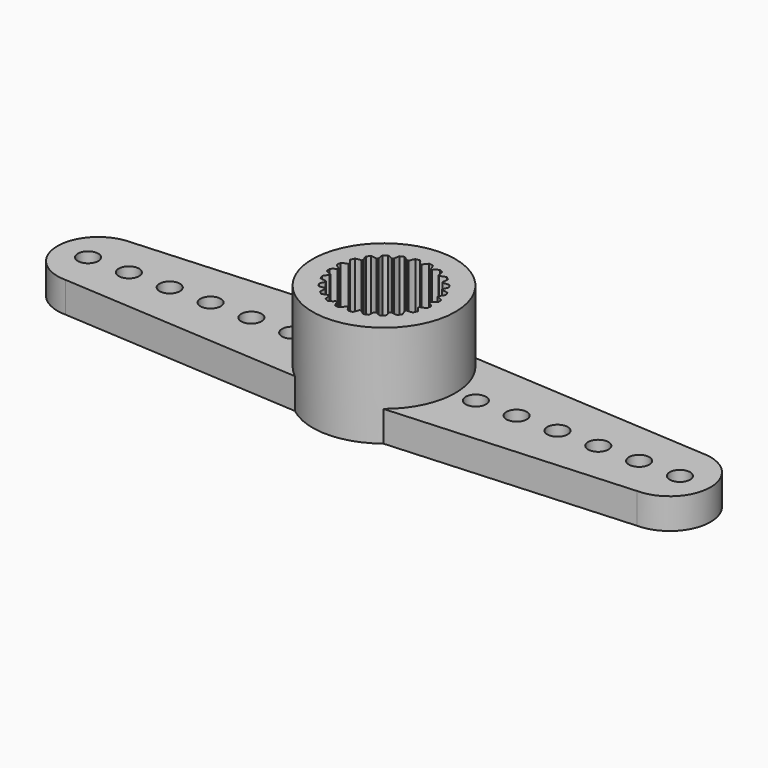
from build123d import *

# Parameters (mm, degrees)
F0_R     = 0.5
F0_R_2   = 1
F1_DEPTH = 1.5
F2_DEPTH = 5
F3_R     = 2.375
F4_DEPTH = 1
F6_DEPTH = 2.75


# Not quite as in the source:
# - a feature names something its author has since deleted; it is built from what else it names


with BuildPart() as f1:
    # F0 (on Top) → F1 (new body)
    with BuildSketch(Plane.XY):
        with BuildLine():
            ThreePointArc((-2.1650635095, -2.75), (-3.5, 0), (-2.1650635095, 2.75))
            Line((-2.1650635095, 2.75), (-14, 2))
            ThreePointArc((-14, 2), (-12.5857864376, 1.4142135624), (-12, 0))
            ThreePointArc((-12, 0), (-12.5857864376, -1.4142135624), (-14, -2))
            Line((-14, -2), (-2.1650635095, -2.75))
        make_face()
        with Locations((-10.5, 0)):
            Circle(F0_R, mode=Mode.SUBTRACT)
        with Locations((-8.5, 0)):
            Circle(F0_R, mode=Mode.SUBTRACT)
        with Locations((-6.5, 0)):
            Circle(F0_R, mode=Mode.SUBTRACT)
        with Locations((-4.5, 0)):
            Circle(F0_R, mode=Mode.SUBTRACT)
        with BuildLine():
            ThreePointArc((-2.1650635095, -2.75), (1.5284432794, -3.148628454), (3.5, 0))
            ThreePointArc((3.5, 0), (1.5284432794, 3.148628454), (-2.1650635095, 2.75))
            ThreePointArc((-2.1650635095, 2.75), (-3.5, 0), (-2.1650635095, -2.75))
        make_face()
        Circle(F0_R_2, mode=Mode.SUBTRACT)
        with BuildLine():
            ThreePointArc((-12, 0), (-12.5857864376, 1.4142135624), (-14, 2))
            ThreePointArc((-14, 2), (-16, 0), (-14, -2))
            ThreePointArc((-14, -2), (-12.5857864376, -1.4142135624), (-12, 0))
        make_face()
        with Locations((-14.5, 0)):
            Circle(F0_R, mode=Mode.SUBTRACT)
        with Locations((-12.5, 0)):
            Circle(F0_R, mode=Mode.SUBTRACT)
    extrude(amount=F1_DEPTH)

    # F0 (on Top) → F2 (join)
    with BuildSketch(Plane.XY):
        with BuildLine():
            ThreePointArc((-2.1650635095, -2.75), (1.5284432794, -3.148628454), (3.5, 0))
            ThreePointArc((3.5, 0), (1.5284432794, 3.148628454), (-2.1650635095, 2.75))
            ThreePointArc((-2.1650635095, 2.75), (-3.5, 0), (-2.1650635095, -2.75))
        make_face()
        Circle(F0_R_2, mode=Mode.SUBTRACT)
    extrude(amount=F2_DEPTH)

    # F3 (on face) → F4 (cut)
    with BuildSketch(Plane.XY):
        Circle(F3_R)
    extrude(amount=F4_DEPTH, mode=Mode.SUBTRACT)

    # F5 (on face) → F6 (cut)
    with BuildSketch(Plane.XY.offset(5)):
        with BuildLine():
            ThreePointArc((2.2496444163, -0.04), (2.2499111023, -0.0200007902), (2.25, 0))
            ThreePointArc((2.25, 0), (2.2499111023, 0.0200007902), (2.2496444163, 0.04))
            ThreePointArc((2.2496444163, 0.04), (2.2307509381, 0.2936839325), (2.1833424035, 0.5436137866))
            ThreePointArc((2.1833424035, 0.5436137866), (2.1733331092, 0.5823428515), (2.1626368799, 0.6208878527))
            ThreePointArc((2.1626368799, 0.6208878527), (2.0787289482, 0.8610377228), (1.968249214, 1.090181192))
            ThreePointArc((1.968249214, 1.090181192), (1.9485571585, 1.125), (1.928249214, 1.1594632243))
            ThreePointArc((1.928249214, 1.1594632243), (1.7850450157, 1.3697132153), (1.6190230933, 1.5624545508))
            ThreePointArc((1.6190230933, 1.5624545508), (1.5909902577, 1.5909902577), (1.5624545508, 1.6190230933))
            ThreePointArc((1.5624545508, 1.6190230933), (1.3697132153, 1.7850450157), (1.1594632243, 1.928249214))
            ThreePointArc((1.1594632243, 1.928249214), (1.125, 1.9485571585), (1.090181192, 1.968249214))
            ThreePointArc((1.090181192, 1.968249214), (0.8610377228, 2.0787289482), (0.6208878527, 2.1626368799))
            ThreePointArc((0.6208878527, 2.1626368799), (0.5823428515, 2.1733331092), (0.5436137866, 2.1833424035))
            ThreePointArc((0.5436137866, 2.1833424035), (0.2936839325, 2.2307509381), (0.04, 2.2496444163))
            ThreePointArc((0.04, 2.2496444163), (0, 2.25), (-0.04, 2.2496444163))
            ThreePointArc((-0.04, 2.2496444163), (-0.2936839325, 2.2307509381), (-0.5436137866, 2.1833424035))
            ThreePointArc((-0.5436137866, 2.1833424035), (-0.5823428515, 2.1733331092), (-0.6208878527, 2.1626368799))
            ThreePointArc((-0.6208878527, 2.1626368799), (-0.8610377228, 2.0787289482), (-1.090181192, 1.968249214))
            ThreePointArc((-1.090181192, 1.968249214), (-1.125, 1.9485571585), (-1.1594632243, 1.928249214))
            ThreePointArc((-1.1594632243, 1.928249214), (-1.3697132153, 1.7850450157), (-1.5624545508, 1.6190230933))
            ThreePointArc((-1.5624545508, 1.6190230933), (-1.5909902577, 1.5909902577), (-1.6190230933, 1.5624545508))
            ThreePointArc((-1.6190230933, 1.5624545508), (-1.7850450157, 1.3697132153), (-1.928249214, 1.1594632243))
            ThreePointArc((-1.928249214, 1.1594632243), (-1.9485571585, 1.125), (-1.968249214, 1.090181192))
            ThreePointArc((-1.968249214, 1.090181192), (-2.0787289482, 0.8610377228), (-2.1626368799, 0.6208878527))
            ThreePointArc((-2.1626368799, 0.6208878527), (-2.1733331092, 0.5823428515), (-2.1833424035, 0.5436137866))
            ThreePointArc((-2.1833424035, 0.5436137866), (-2.2307509381, 0.2936839325), (-2.2496444163, 0.04))
            ThreePointArc((-2.2496444163, 0.04), (-2.25, 0), (-2.2496444163, -0.04))
            ThreePointArc((-2.2496444163, -0.04), (-2.2307509381, -0.2936839325), (-2.1833424035, -0.5436137866))
            ThreePointArc((-2.1833424035, -0.5436137866), (-2.1733331092, -0.5823428515), (-2.1626368799, -0.6208878527))
            ThreePointArc((-2.1626368799, -0.6208878527), (-2.0787289482, -0.8610377228), (-1.968249214, -1.090181192))
            ThreePointArc((-1.968249214, -1.090181192), (-1.9485571585, -1.125), (-1.928249214, -1.1594632243))
            ThreePointArc((-1.928249214, -1.1594632243), (-1.7850450157, -1.3697132153), (-1.6190230933, -1.5624545508))
            ThreePointArc((-1.6190230933, -1.5624545508), (-1.5909902577, -1.5909902577), (-1.5624545508, -1.6190230933))
            ThreePointArc((-1.5624545508, -1.6190230933), (-1.3697132153, -1.7850450157), (-1.1594632243, -1.928249214))
            ThreePointArc((-1.1594632243, -1.928249214), (-1.125, -1.9485571585), (-1.090181192, -1.968249214))
            ThreePointArc((-1.090181192, -1.968249214), (-0.8610377228, -2.0787289482), (-0.6208878527, -2.1626368799))
            ThreePointArc((-0.6208878527, -2.1626368799), (-0.5823428515, -2.1733331092), (-0.5436137866, -2.1833424035))
            ThreePointArc((-0.5436137866, -2.1833424035), (-0.2936839325, -2.2307509381), (-0.04, -2.2496444163))
            ThreePointArc((-0.04, -2.2496444163), (0, -2.25), (0.04, -2.2496444163))
            ThreePointArc((0.04, -2.2496444163), (0.2936839325, -2.2307509381), (0.5436137866, -2.1833424035))
            ThreePointArc((0.5436137866, -2.1833424035), (0.5823428515, -2.1733331092), (0.6208878527, -2.1626368799))
            ThreePointArc((0.6208878527, -2.1626368799), (0.8610377228, -2.0787289482), (1.090181192, -1.968249214))
            ThreePointArc((1.090181192, -1.968249214), (1.125, -1.9485571585), (1.1594632243, -1.928249214))
            ThreePointArc((1.1594632243, -1.928249214), (1.3697132153, -1.7850450157), (1.5624545508, -1.6190230933))
            ThreePointArc((1.5624545508, -1.6190230933), (1.5909902577, -1.5909902577), (1.6190230933, -1.5624545508))
            ThreePointArc((1.6190230933, -1.5624545508), (1.7850450157, -1.3697132153), (1.928249214, -1.1594632243))
            ThreePointArc((1.928249214, -1.1594632243), (1.9485571585, -1.125), (1.968249214, -1.090181192))
            ThreePointArc((1.968249214, -1.090181192), (2.0787289482, -0.8610377228), (2.1626368799, -0.6208878527))
            ThreePointArc((2.1626368799, -0.6208878527), (2.1733331092, -0.5823428515), (2.1833424035, -0.5436137866))
            ThreePointArc((2.1833424035, -0.5436137866), (2.2307509381, -0.2936839325), (2.2496444163, -0.04))
        make_face()
        with BuildLine():
            ThreePointArc((2.1833424035, 0.5436137866), (2.2307509381, 0.2936839325), (2.2496444163, 0.04))
            ThreePointArc((2.2496444163, 0.04), (2.376347735, 0.1239325273), (2.4898544134, 0.225))
            ThreePointArc((2.4898544134, 0.225), (2.47674458, 0.3260696098), (2.4632489668, 0.4270884308))
            ThreePointArc((2.4632489668, 0.4270884308), (2.3313772515, 0.5047639091), (2.1833424035, 0.5436137866))
        make_face()
        with BuildLine():
            ThreePointArc((2.4898544134, -0.225), (2.382580011, -0.115840338), (2.2496444163, -0.04))
            ThreePointArc((2.2496444163, -0.04), (2.2307509381, -0.2936839325), (2.1833424035, -0.5436137866))
            ThreePointArc((2.1833424035, -0.5436137866), (2.3274517478, -0.4953344228), (2.4632489668, -0.4270884308))
            ThreePointArc((2.4632489668, -0.4270884308), (2.47674458, -0.3260696098), (2.4898544134, -0.225))
        make_face()
        with BuildLine():
            ThreePointArc((1.968249214, 1.090181192), (2.0787289482, 0.8610377228), (2.1626368799, 0.6208878527))
            ThreePointArc((2.1626368799, 0.6208878527), (2.2632995511, 0.7347536804), (2.3467803965, 0.8617550526))
            ThreePointArc((2.3467803965, 0.8617550526), (2.3079585298, 0.9559877245), (2.2687771737, 1.0500714909))
            ThreePointArc((2.2687771737, 1.0500714909), (2.1212949851, 1.09096933), (1.968249214, 1.090181192))
        make_face()
        with BuildLine():
            ThreePointArc((2.3467803965, -0.8617550526), (2.2714138802, -0.7285502576), (2.1626368799, -0.6208878527))
            ThreePointArc((2.1626368799, -0.6208878527), (2.0787289482, -0.8610377228), (1.968249214, -1.090181192))
            ThreePointArc((1.968249214, -1.090181192), (2.1199437704, -1.0808451505), (2.2687771737, -1.0500714909))
            ThreePointArc((2.2687771737, -1.0500714909), (2.3079585298, -0.9559877245), (2.3467803965, -0.8617550526))
        make_face()
        with BuildLine():
            ThreePointArc((1.6190230933, 1.5624545508), (1.7850450157, 1.3697132153), (1.928249214, 1.1594632243))
            ThreePointArc((1.928249214, 1.1594632243), (1.9960112431, 1.2955025845), (2.0437771737, 1.4397829226))
            ThreePointArc((2.0437771737, 1.4397829226), (1.98188892, 1.5207568555), (1.9196919657, 1.6014939141))
            ThreePointArc((1.9196919657, 1.6014939141), (1.7666499711, 1.602826994), (1.6190230933, 1.5624545508))
        make_face()
        with BuildLine():
            ThreePointArc((2.0437771737, -1.4397829226), (2.0054546471, -1.291610681), (1.928249214, -1.1594632243))
            ThreePointArc((1.928249214, -1.1594632243), (1.7850450157, -1.3697132153), (1.6190230933, -1.5624545508))
            ThreePointArc((1.6190230933, -1.5624545508), (1.7679651283, -1.5926980674), (1.9196919657, -1.6014939141))
            ThreePointArc((1.9196919657, -1.6014939141), (1.98188892, -1.5207568555), (2.0437771737, -1.4397829226))
        make_face()
        with BuildLine():
            ThreePointArc((1.1594632243, 1.928249214), (1.3697132153, 1.7850450157), (1.5624545508, 1.6190230933))
            ThreePointArc((1.5624545508, 1.6190230933), (1.5926980674, 1.7679651283), (1.6014939141, 1.9196919657))
            ThreePointArc((1.6014939141, 1.9196919657), (1.5207568555, 1.98188892), (1.4397829226, 2.0437771737))
            ThreePointArc((1.4397829226, 2.0437771737), (1.291610681, 2.0054546471), (1.1594632243, 1.928249214))
        make_face()
        with BuildLine():
            ThreePointArc((1.6014939141, -1.9196919657), (1.602826994, -1.7666499711), (1.5624545508, -1.6190230933))
            ThreePointArc((1.5624545508, -1.6190230933), (1.3697132153, -1.7850450157), (1.1594632243, -1.928249214))
            ThreePointArc((1.1594632243, -1.928249214), (1.2955025845, -1.9960112431), (1.4397829226, -2.0437771737))
            ThreePointArc((1.4397829226, -2.0437771737), (1.5207568555, -1.98188892), (1.6014939141, -1.9196919657))
        make_face()
        with BuildLine():
            ThreePointArc((0.6208878527, 2.1626368799), (0.8610377228, 2.0787289482), (1.090181192, 1.968249214))
            ThreePointArc((1.090181192, 1.968249214), (1.0808451505, 2.1199437704), (1.0500714909, 2.2687771737))
            ThreePointArc((1.0500714909, 2.2687771737), (0.9559877245, 2.3079585298), (0.8617550526, 2.3467803965))
            ThreePointArc((0.8617550526, 2.3467803965), (0.7285502576, 2.2714138802), (0.6208878527, 2.1626368799))
        make_face()
        with BuildLine():
            ThreePointArc((1.0500714909, -2.2687771737), (1.09096933, -2.1212949851), (1.090181192, -1.968249214))
            ThreePointArc((1.090181192, -1.968249214), (0.8610377228, -2.0787289482), (0.6208878527, -2.1626368799))
            ThreePointArc((0.6208878527, -2.1626368799), (0.7347536804, -2.2632995511), (0.8617550526, -2.3467803965))
            ThreePointArc((0.8617550526, -2.3467803965), (0.9559877245, -2.3079585298), (1.0500714909, -2.2687771737))
        make_face()
        with BuildLine():
            ThreePointArc((0.04, 2.2496444163), (0.2936839325, 2.2307509381), (0.5436137866, 2.1833424035))
            ThreePointArc((0.5436137866, 2.1833424035), (0.4953344228, 2.3274517478), (0.4270884308, 2.4632489668))
            ThreePointArc((0.4270884308, 2.4632489668), (0.3260696098, 2.47674458), (0.225, 2.4898544134))
            ThreePointArc((0.225, 2.4898544134), (0.115840338, 2.382580011), (0.04, 2.2496444163))
        make_face()
        with BuildLine():
            ThreePointArc((0.4270884308, -2.4632489668), (0.5047639091, -2.3313772515), (0.5436137866, -2.1833424035))
            ThreePointArc((0.5436137866, -2.1833424035), (0.2936839325, -2.2307509381), (0.04, -2.2496444163))
            ThreePointArc((0.04, -2.2496444163), (0.1239325273, -2.376347735), (0.225, -2.4898544134))
            ThreePointArc((0.225, -2.4898544134), (0.3260696098, -2.47674458), (0.4270884308, -2.4632489668))
        make_face()
        with BuildLine():
            ThreePointArc((-0.5436137866, 2.1833424035), (-0.2936839325, 2.2307509381), (-0.04, 2.2496444163))
            ThreePointArc((-0.04, 2.2496444163), (-0.1239325273, 2.376347735), (-0.225, 2.4898544134))
            ThreePointArc((-0.225, 2.4898544134), (-0.3260696098, 2.47674458), (-0.4270884308, 2.4632489668))
            ThreePointArc((-0.4270884308, 2.4632489668), (-0.5047639091, 2.3313772515), (-0.5436137866, 2.1833424035))
        make_face()
        with BuildLine():
            ThreePointArc((-0.225, -2.4898544134), (-0.115840338, -2.382580011), (-0.04, -2.2496444163))
            ThreePointArc((-0.04, -2.2496444163), (-0.2936839325, -2.2307509381), (-0.5436137866, -2.1833424035))
            ThreePointArc((-0.5436137866, -2.1833424035), (-0.4953344228, -2.3274517478), (-0.4270884308, -2.4632489668))
            ThreePointArc((-0.4270884308, -2.4632489668), (-0.3260696098, -2.47674458), (-0.225, -2.4898544134))
        make_face()
        with BuildLine():
            ThreePointArc((-1.090181192, 1.968249214), (-0.8610377228, 2.0787289482), (-0.6208878527, 2.1626368799))
            ThreePointArc((-0.6208878527, 2.1626368799), (-0.7347536804, 2.2632995511), (-0.8617550526, 2.3467803965))
            ThreePointArc((-0.8617550526, 2.3467803965), (-0.9559877245, 2.3079585298), (-1.0500714909, 2.2687771737))
            ThreePointArc((-1.0500714909, 2.2687771737), (-1.09096933, 2.1212949851), (-1.090181192, 1.968249214))
        make_face()
        with BuildLine():
            ThreePointArc((-0.8617550526, -2.3467803965), (-0.7285502576, -2.2714138802), (-0.6208878527, -2.1626368799))
            ThreePointArc((-0.6208878527, -2.1626368799), (-0.8610377228, -2.0787289482), (-1.090181192, -1.968249214))
            ThreePointArc((-1.090181192, -1.968249214), (-1.0808451505, -2.1199437704), (-1.0500714909, -2.2687771737))
            ThreePointArc((-1.0500714909, -2.2687771737), (-0.9559877245, -2.3079585298), (-0.8617550526, -2.3467803965))
        make_face()
        with BuildLine():
            ThreePointArc((-1.5624545508, 1.6190230933), (-1.3697132153, 1.7850450157), (-1.1594632243, 1.928249214))
            ThreePointArc((-1.1594632243, 1.928249214), (-1.2955025845, 1.9960112431), (-1.4397829226, 2.0437771737))
            ThreePointArc((-1.4397829226, 2.0437771737), (-1.5207568555, 1.98188892), (-1.6014939141, 1.9196919657))
            ThreePointArc((-1.6014939141, 1.9196919657), (-1.602826994, 1.7666499711), (-1.5624545508, 1.6190230933))
        make_face()
        with BuildLine():
            ThreePointArc((-1.4397829226, -2.0437771737), (-1.291610681, -2.0054546471), (-1.1594632243, -1.928249214))
            ThreePointArc((-1.1594632243, -1.928249214), (-1.3697132153, -1.7850450157), (-1.5624545508, -1.6190230933))
            ThreePointArc((-1.5624545508, -1.6190230933), (-1.5926980674, -1.7679651283), (-1.6014939141, -1.9196919657))
            ThreePointArc((-1.6014939141, -1.9196919657), (-1.5207568555, -1.98188892), (-1.4397829226, -2.0437771737))
        make_face()
        with BuildLine():
            ThreePointArc((-1.928249214, 1.1594632243), (-1.7850450157, 1.3697132153), (-1.6190230933, 1.5624545508))
            ThreePointArc((-1.6190230933, 1.5624545508), (-1.7679651283, 1.5926980674), (-1.9196919657, 1.6014939141))
            ThreePointArc((-1.9196919657, 1.6014939141), (-1.98188892, 1.5207568555), (-2.0437771737, 1.4397829226))
            ThreePointArc((-2.0437771737, 1.4397829226), (-2.0054546471, 1.291610681), (-1.928249214, 1.1594632243))
        make_face()
        with BuildLine():
            ThreePointArc((-1.9196919657, -1.6014939141), (-1.7666499711, -1.602826994), (-1.6190230933, -1.5624545508))
            ThreePointArc((-1.6190230933, -1.5624545508), (-1.7850450157, -1.3697132153), (-1.928249214, -1.1594632243))
            ThreePointArc((-1.928249214, -1.1594632243), (-1.9960112431, -1.2955025845), (-2.0437771737, -1.4397829226))
            ThreePointArc((-2.0437771737, -1.4397829226), (-1.98188892, -1.5207568555), (-1.9196919657, -1.6014939141))
        make_face()
        with BuildLine():
            ThreePointArc((-2.1626368799, 0.6208878527), (-2.0787289482, 0.8610377228), (-1.968249214, 1.090181192))
            ThreePointArc((-1.968249214, 1.090181192), (-2.1199437704, 1.0808451505), (-2.2687771737, 1.0500714909))
            ThreePointArc((-2.2687771737, 1.0500714909), (-2.3079585298, 0.9559877245), (-2.3467803965, 0.8617550526))
            ThreePointArc((-2.3467803965, 0.8617550526), (-2.2714138802, 0.7285502576), (-2.1626368799, 0.6208878527))
        make_face()
        with BuildLine():
            ThreePointArc((-2.2687771737, -1.0500714909), (-2.1212949851, -1.09096933), (-1.968249214, -1.090181192))
            ThreePointArc((-1.968249214, -1.090181192), (-2.0787289482, -0.8610377228), (-2.1626368799, -0.6208878527))
            ThreePointArc((-2.1626368799, -0.6208878527), (-2.2632995511, -0.7347536804), (-2.3467803965, -0.8617550526))
            ThreePointArc((-2.3467803965, -0.8617550526), (-2.3079585298, -0.9559877245), (-2.2687771737, -1.0500714909))
        make_face()
        with BuildLine():
            ThreePointArc((-2.2496444163, 0.04), (-2.2307509381, 0.2936839325), (-2.1833424035, 0.5436137866))
            ThreePointArc((-2.1833424035, 0.5436137866), (-2.3274517478, 0.4953344228), (-2.4632489668, 0.4270884308))
            ThreePointArc((-2.4632489668, 0.4270884308), (-2.47674458, 0.3260696098), (-2.4898544134, 0.225))
            ThreePointArc((-2.4898544134, 0.225), (-2.382580011, 0.115840338), (-2.2496444163, 0.04))
        make_face()
        with BuildLine():
            ThreePointArc((-2.4632489668, -0.4270884308), (-2.3313772515, -0.5047639091), (-2.1833424035, -0.5436137866))
            ThreePointArc((-2.1833424035, -0.5436137866), (-2.2307509381, -0.2936839325), (-2.2496444163, -0.04))
            ThreePointArc((-2.2496444163, -0.04), (-2.376347735, -0.1239325273), (-2.4898544134, -0.225))
            ThreePointArc((-2.4898544134, -0.225), (-2.47674458, -0.3260696098), (-2.4632489668, -0.4270884308))
        make_face()
    extrude(amount=-F6_DEPTH, mode=Mode.SUBTRACT)

    # F7: F1 across plane


with BuildPart() as f1_1:
    add(f1.part)
    add(f1.part.mirror(Plane.YZ))


solid = f1_1.part
